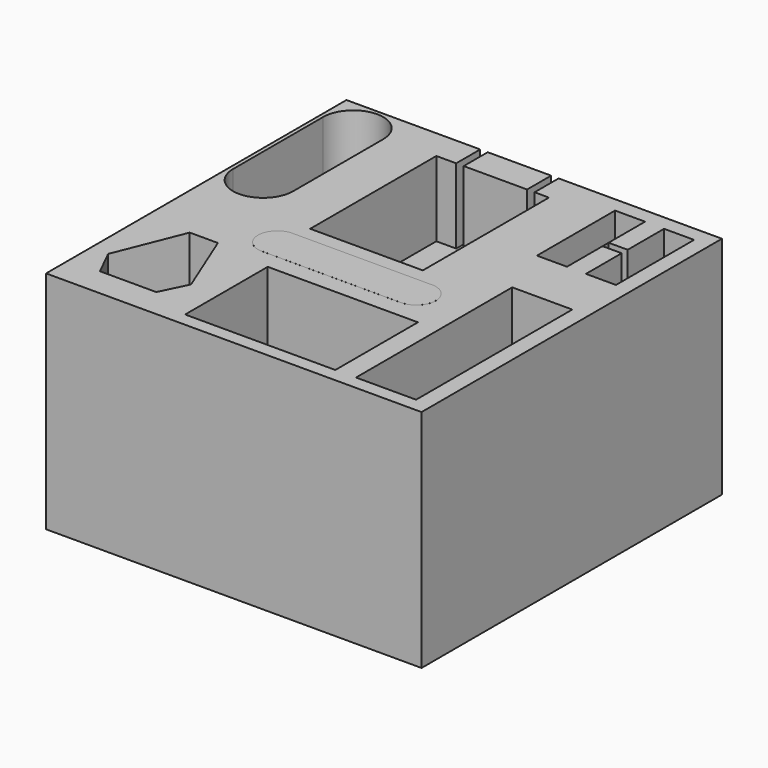
from build123d import *

# Parameters (mm, degrees)
F1_W        = 15544.8
F1_H        = 6096
F7_DEPTH    = 182880
F4_W        = 6096
F4_H        = 24384
F0_W        = 24384
F0_H        = 79248
F0_W_2      = 3048
F0_H_2      = 27432
F5_W        = 121920
F5_H        = 83820
F3_W        = 48768.0000000001
F3_H        = 158496
F8_DEPTH    = 60960
F7_FACE_W   = 15544.8
F7_FACE_H   = 6096
F7_FACE_W_2 = 24384
F7_FACE_H_2 = 79248
F7_FACE_W_3 = 48768.0000000001
F7_FACE_H_3 = 158496
F7_FACE_W_4 = 121920
F7_FACE_H_4 = 83820
F9_DEPTH    = 60960
F17_DEPTH   = 30.48


# Not quite as in the source:
# - the program builds the solid bodies; features that only make, move or delete a surface that nothing else refers to are left out


with BuildPart() as f7:
    # F1 (on face) → F7 (new body)
    with BuildSketch(Plane.XY):
        with Locations((107550.465918614, 100174.9229431152)):
            Rectangle(F1_W, F1_H)
    extrude(amount=F7_DEPTH)


with BuildPart() as f7b:
    # F6 (on face) → F7, piece 2 (new body)
    with BuildSketch(Plane.XY):
        Polygon((-138384.5689090631, -106939.4663491444), (-127551.5013376337, -128784.9259001094), (-81831.5013376337, -128784.9259001094), (-71159.4495909771, -106860.3559495566), (-93440.3353419917, -51758.629786484), (-116300.3353419917, -51758.629786484), align=None)
    extrude(amount=F7_DEPTH)


with BuildPart() as f7c:
    # F4 (on face) → F7, piece 3 (new body)
    with BuildSketch(Plane.XY):
        Polygon((-43811.408996582, 128016), (-59924.1409301758, 128016), (-59924.1409301758, 0), (31515.8590698242, 0), (31515.8590698242, 128016), (19836.6167984009, 128016), (13740.6167984009, 128016), (-37715.408996582, 128016), align=None)
        with Locations((-40763.408996582, 140208)):
            Rectangle(F4_W, F4_H)
        with Locations((16788.6167984009, 140208)):
            Rectangle(F4_W, F4_H)
    extrude(amount=F7_DEPTH)


with BuildPart() as f7d:
    # F0 (on Top) → F7, piece 4 (new body)
    with BuildSketch(Plane.XY):
        Polygon((152400, -152400), (152400, 152400), (-149352, 152400), (-149352, 124968), (-152400.0000000001, 124968), (-152400, -152400), align=None)
        with BuildLine():
            Line((-149352, 33528), (-149352, 124968))
            ThreePointArc((-149352, 124968), (-142210.0917524528, 142210.0917524528), (-124968, 149352))
            ThreePointArc((-124968, 149352), (-107725.9082475473, 142210.0917524527), (-100584.0000000001, 124968))
            Line((-100584, 124968), (-100584, 33528))
            ThreePointArc((-100584, 33528), (-124968, 9144), (-149352, 33528))
        make_face(mode=Mode.SUBTRACT)
        with Locations((127422.9112548828, 100502.7536621094)):
            Rectangle(F0_W, F0_H, mode=Mode.SUBTRACT)
        with Locations((-150876, 138684)):
            Rectangle(F0_W_2, F0_H_2)
    extrude(amount=F7_DEPTH)


with BuildPart() as f7e:
    # F5 (on face) → F7, piece 5 (new body)
    with BuildSketch(Plane.XY):
        with Locations((12639.0037536621, -99496.3893408147)):
            Rectangle(F5_W, F5_H)
    extrude(amount=F7_DEPTH)


with BuildPart() as f7f:
    # F2 (on face) → F7, piece 6 (new body)
    with BuildSketch(Plane.XY):
        Polygon((99736.4994638944, 100631.8702697754), (99736.4994638944, 140255.8702697754), (75352.4994638944, 140255.8702697754), (75352.4994638944, 61007.8702697754), (99736.4994638944, 61007.8702697754), (99736.4994638944, 90581.0760098918), align=None)
    extrude(amount=F7_DEPTH)


with BuildPart() as f7g:
    # F3 (on face) → F7, piece 7 (new body)
    with BuildSketch(Plane.XY):
        with Locations((114696.2353164215, -62032.543182373)):
            Rectangle(F3_W, F3_H)
    extrude(amount=F7_DEPTH)


with BuildPart() as f8_tool:
    # F8 (cut): a face of the model
    f8_faces = [f7c.part.faces().sort_by_distance(p)[0] for p in [
        (-14149.2370334306, 65895.306501548, 182880),
    ]]
    extrude(f8_faces, amount=-F8_DEPTH)


with BuildPart() as f7c_1:
    add(f7c.part)

    # F8: cut by f8_tool
    add(f8_tool.part, mode=Mode.SUBTRACT)


with BuildPart() as f7d_1:
    add(f7d.part)

    # F8: cut by f8_tool
    add(f8_tool.part, mode=Mode.SUBTRACT)


with BuildPart() as f9_tool:
    # F7_face (on face) → F9 (new body)
    with BuildSketch(Plane(origin=(-14149.2370334306, 65895.306501548, 182880), x_dir=(1, 0, 0), z_dir=(0, 0, 1))):
        with Locations((121699.7029520446, 34279.6164415673)):
            Rectangle(F7_FACE_W, F7_FACE_H)
        Polygon((-124235.3318756325, -172834.7728506924), (-113402.2643042031, -194680.2324016574), (-67682.2643042031, -194680.2324016574), (-57010.2125575465, -172755.6624511046), (-79291.0983085611, -117653.936288032), (-102151.0983085611, -117653.936288032), align=None)
        with Locations((101693.736497325, 34736.5637682274)):
            Rectangle(F7_FACE_W_2, F7_FACE_H_2)
        with Locations((128845.4723498522, -127927.849683921)):
            Rectangle(F7_FACE_W_3, F7_FACE_H_3)
        with Locations((26788.2407870928, -165391.6958423627)):
            Rectangle(F7_FACE_W_4, F7_FACE_H_4)
    extrude(amount=-F9_DEPTH)


with BuildPart() as f7_1:
    add(f7.part)

    # F9: cut by f9_tool
    add(f9_tool.part, mode=Mode.SUBTRACT)


with BuildPart() as f7b_1:
    add(f7b.part)

    # F9: cut by f9_tool
    add(f9_tool.part, mode=Mode.SUBTRACT)


with BuildPart() as f7d_2:
    add(f7d_1.part)

    # F9: cut by f9_tool
    add(f9_tool.part, mode=Mode.SUBTRACT)

    # F16 (on face) → F17 (join)
    with BuildSketch(Plane.XY.offset(182880)):
        with BuildLine():
            ThreePointArc((-66410.8023529053, -11879.8866271973), (-80244.7849895234, -28445.0095732925), (-64535.0865011215, -43243.2441711426))
            Line((-64535.0865011215, -43243.2441711426), (48240.9134988785, -43243.2441711426))
            ThreePointArc((48240.9134988785, -43243.2441711426), (63950.6119872804, -26565.9422291696), (46365.1976470947, -11879.8866271973))
            Line((46365.1976470947, -11879.8866271973), (-66410.8023529053, -11879.8866271973))
        make_face()
    extrude(amount=F17_DEPTH)


with BuildPart() as f7e_1:
    add(f7e.part)

    # F9: cut by f9_tool
    add(f9_tool.part, mode=Mode.SUBTRACT)


with BuildPart() as f7f_1:
    add(f7f.part)

    # F9: cut by f9_tool
    add(f9_tool.part, mode=Mode.SUBTRACT)


with BuildPart() as f7g_1:
    add(f7g.part)

    # F9: cut by f9_tool
    add(f9_tool.part, mode=Mode.SUBTRACT)


solid = Compound([f7c_1.part, f7_1.part, f7b_1.part, f7d_2.part, f7e_1.part, f7f_1.part, f7g_1.part])
